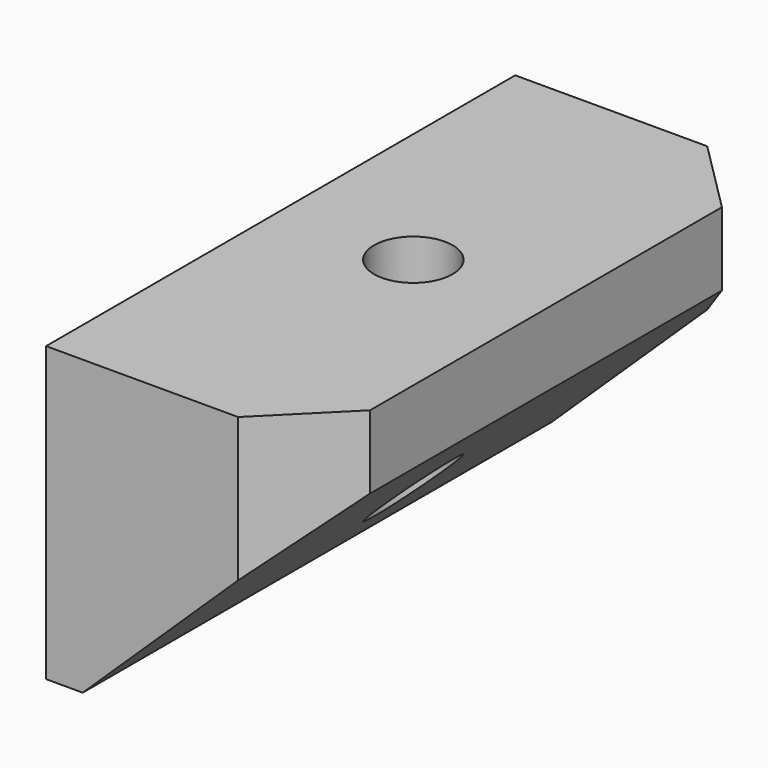
from build123d import *

# Parameters (mm, degrees)
F0_W        = 22.987
F0_H        = 25.4
F1_DEPTH    = 25.4
F3_D        = 6.8
F4_SIZE     = 6.35
F5_SIZE     = 6.35
F6_T1_DEPTH = 140.0532259942


# Not quite as in the source:
# - a fillet or chamfer that OpenCascade refuses, or shapes differently, is made with other operations: its cross-section is extruded or revolved along the edge and cut away or added


with BuildPart() as f1:
    # F0 (on Front) → F1 (new body, symmetric)
    with BuildSketch(Plane.XZ):
        Rectangle(F0_W, F0_H)
    extrude(amount=F1_DEPTH, both=True)

    # F3 (through all)
    with Locations(Plane.XY.offset(12.7)):
        with Locations((0, 0)):
            Hole(F3_D / 2)

    # F4
    f4_edges = [f1.edges().sort_by_distance(p)[0] for p in [
        (11.4935, -25.4, 0),
    ]]
    chamfer(f4_edges, length=F4_SIZE)

    # F5
    f5_edges = [f1.edges().sort_by_distance(p)[0] for p in [
        (11.4935, 25.4, 0),
    ]]
    chamfer(f5_edges, length=F5_SIZE)

    # F6: chamfer of 19.05 x 19.812 on 1 edges, made by hand

    # F6_s2 → F6_t1 (cut)
    with BuildSketch(Plane.XZ.offset(-70.0266129971)):
        Polygon((11.4935, 6.35), (-8.3185, -12.7), (11.4935, -12.7), align=None)
    extrude(amount=F6_T1_DEPTH, mode=Mode.SUBTRACT)


solid = f1.part
